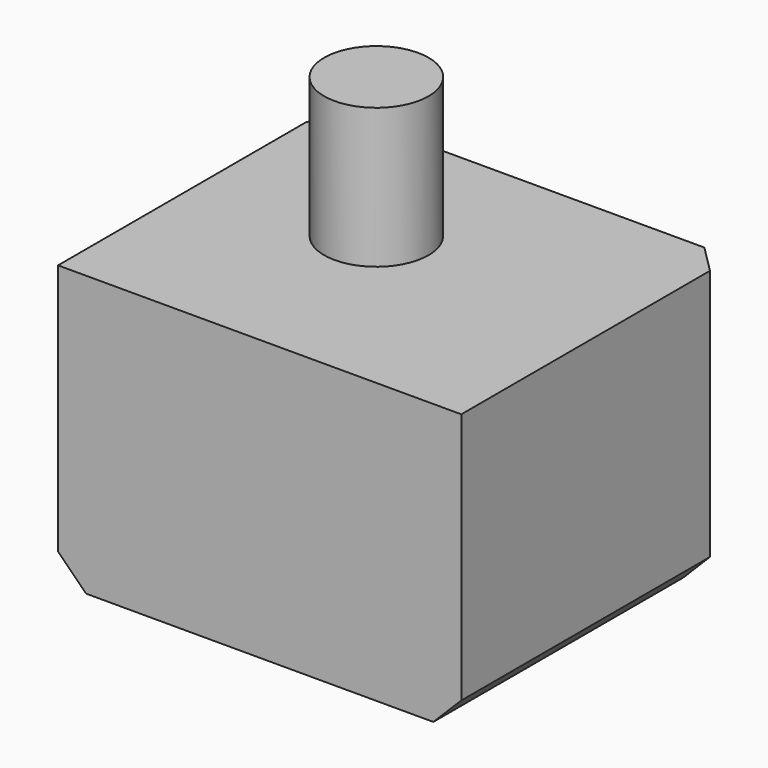
from build123d import *

# Parameters (mm, degrees)
F0_W     = 36.594145
F0_H     = 61.4954829216
F1_DEPTH = 25.4
F2_DEPTH = 25.4
F3_R     = 5.08
F4_SIZE  = 5.07999
F5_R     = 9.4762574088
F6_DEPTH = 25.4


# Not quite as in the source:
# - a fillet or chamfer is up to 0.001 mm smaller than in the source, because OpenCascade refuses the exact size


with BuildPart() as f1:
    # F0 (on Top) → F1 (new body)
    with BuildSketch(Plane.XY):
        with Locations((-12.8837414086, -3.4645497799)):
            Rectangle(F0_W, F0_H)
        with Locations((23.7104035914, -3.4645497799)):
            Rectangle(F0_W, F0_H)
    extrude(amount=F1_DEPTH)

    # F2 (add): a face of the model
    f2_faces = [f1.faces().sort_by_distance(p)[0] for p in [
        (5.4133310914, -3.4645497799, 25.4),
    ]]
    extrude(f2_faces, amount=F2_DEPTH)

    # F3
    f3_edges = [f1.edges().sort_by_distance(p)[0] for p in [
        (5.413331, 27.283192, 0),
    ]]
    fillet(f3_edges, radius=F3_R)

    # F4 (size 5.08 in the source; OpenCascade refuses exactly that, so slightly less here)
    f4_edges = [f1.edges().sort_by_distance(p)[0] for p in [
        (-31.180814, 27.283192, 27.94),
        (42.007476, 27.283192, 27.94),
        (42.007476, -6.00455, 0),
    ]]
    chamfer(f4_edges, length=F4_SIZE)

    # F5 (on face) → F6 (join)
    with BuildSketch(Plane.XY.offset(50.8)):
        with Locations((-1.593567431, 1.0238895973)):
            Circle(F5_R)
    extrude(amount=F6_DEPTH)


solid = f1.part
